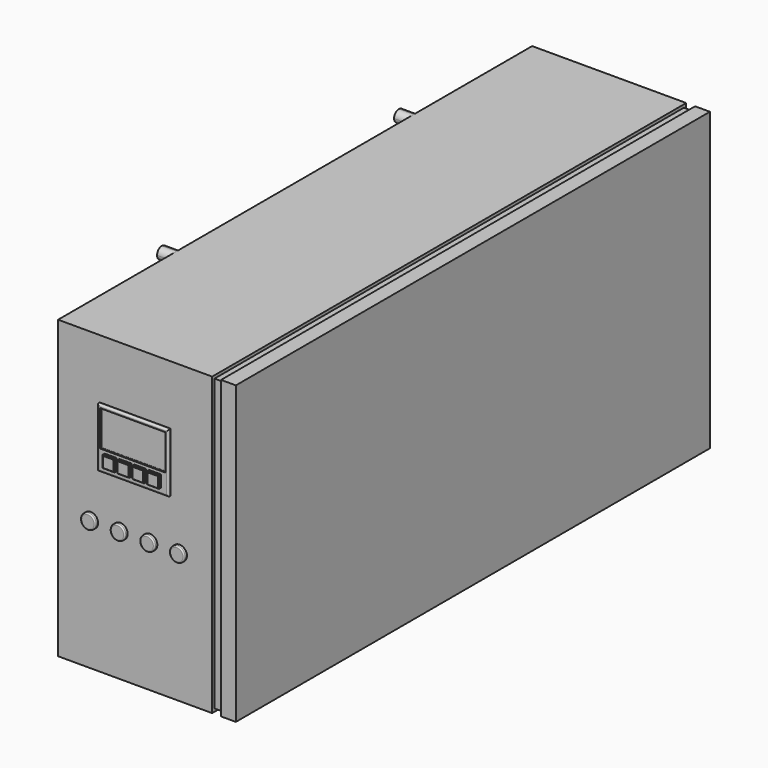
from build123d import *

# Parameters (mm, degrees)
F0_W      = 300
F0_H      = 500
F1_DEPTH  = 1000
F3_W      = 1000
F3_H      = 500
F3_W_2    = 990
F3_H_2    = 490
F4_DEPTH  = 15
F6_DEPTH  = 25
F7_W      = 120
F7_H      = 100
F8_DEPTH  = 5
F9_W      = 20
F9_H      = 20
F10_DEPTH = 5
F11_W     = 110
F11_H     = 60
F12_DEPTH = 2
F14_R     = 12.5
F15_DEPTH = 6
F16_R     = 2
F17_R     = 3
F18_SIZE  = 1
F19_R     = 1


with BuildPart() as f1:
    # F0 (on Front) → F1 (new body)
    with BuildSketch(Plane.XZ):
        with Locations((150, 250)):
            Rectangle(F0_W, F0_H)
    extrude(amount=F1_DEPTH)

    # F3 (on offset) → F4 (cut)
    with BuildSketch(Plane.YZ.offset(275)):
        with Locations((-500, 250)):
            Rectangle(F3_W, F3_H)
        with Locations((-500, 250)):
            Rectangle(F3_W_2, F3_H_2, mode=Mode.SUBTRACT)
    extrude(amount=-F4_DEPTH, mode=Mode.SUBTRACT)

    # F5 (on face) → F6 (join)
    with BuildSketch(Plane(origin=(0, 0, 0), x_dir=(0, -1, 0), z_dir=(-1, 0, 0))):
        with BuildLine():
            ThreePointArc((250.000000113, 500), (242.9289321482, 482.9289322281), (260, 490))
            ThreePointArc((260, 490), (257.0710678518, 497.0710677719), (250.000000113, 500))
        make_face()
        with BuildLine():
            ThreePointArc((260, 10), (242.9289321881, 17.0710678119), (250, 0))
            ThreePointArc((250, 0), (257.0710678119, 2.9289321881), (260, 10))
        make_face()
        with BuildLine():
            ThreePointArc((760, 10), (742.9289321881, 17.0710678119), (750, 0))
            ThreePointArc((750, 0), (757.0710678119, 2.9289321881), (760, 10))
        make_face()
        with BuildLine():
            ThreePointArc((760, 490), (757.0710678119, 497.0710678119), (750, 500))
            ThreePointArc((750, 500), (742.9289321881, 482.9289321881), (760, 490))
        make_face()
    extrude(amount=F6_DEPTH)

    # F7 (on face) → F8 (join)
    with BuildSketch(Plane.XZ.offset(1000)):
        with Locations((130, 350)):
            Rectangle(F7_W, F7_H)
    extrude(amount=F8_DEPTH)

    # F9 (on face) → F10 (join)
    with BuildSketch(Plane.XZ.offset(1005)):
        with Locations((92.5, 320)):
            Rectangle(F9_W, F9_H)
        with Locations((117.5, 320)):
            Rectangle(F9_W, F9_H)
        with Locations((142.5, 320)):
            Rectangle(F9_W, F9_H)
        with Locations((167.5, 320)):
            Rectangle(F9_W, F9_H)
    extrude(amount=F10_DEPTH)

    # F11 (on face) → F12 (cut)
    with BuildSketch(Plane.XZ.offset(1005)):
        with Locations((130, 365)):
            Rectangle(F11_W, F11_H)
    extrude(amount=-F12_DEPTH, mode=Mode.SUBTRACT)

    # F14 (on face) → F15 (join)
    with BuildSketch(Plane.XZ.offset(1000)):
        with Locations((55, 220)):
            Circle(F14_R)
        with Locations((105, 220)):
            Circle(F14_R)
        with Locations((155, 220)):
            Circle(F14_R)
        with Locations((205, 220)):
            Circle(F14_R)
    extrude(amount=F15_DEPTH)

    # F16
    f16_edges = [f1.edges().sort_by_distance(p)[0] for p in [
        (42.5, -1006, 220),
        (92.5, -1006, 220),
        (142.5, -1006, 220),
        (192.5, -1006, 220),
    ]]
    fillet(f16_edges, radius=F16_R)

    # F17
    f17_edges = [f1.edges().sort_by_distance(p)[0] for p in [
        (70, -1005, 350),
        (130, -1005, 300),
        (190, -1005, 350),
        (130, -1005, 400),
    ]]
    fillet(f17_edges, radius=F17_R)

    # F18
    f18_edges = [f1.edges().sort_by_distance(p)[0] for p in [
        (92.5, -1010, 330),
        (82.5, -1010, 320),
        (92.5, -1010, 310),
        (102.5, -1010, 320),
        (117.5, -1010, 330),
        (107.5, -1010, 320),
        (117.5, -1010, 310),
        (127.5, -1010, 320),
        (142.5, -1010, 330),
        (132.5, -1010, 320),
        (142.5, -1010, 310),
        (152.5, -1010, 320),
        (167.5, -1010, 330),
        (157.5, -1010, 320),
        (167.5, -1010, 310),
        (177.5, -1010, 320),
    ]]
    chamfer(f18_edges, length=F18_SIZE)

    # F19
    f19_edges = [f1.edges().sort_by_distance(p)[0] for p in [
        (130, -1003, 395),
        (75, -1003, 365),
        (130, -1003, 335),
        (185, -1003, 365),
    ]]
    fillet(f19_edges, radius=F19_R)


solid = f1.part
